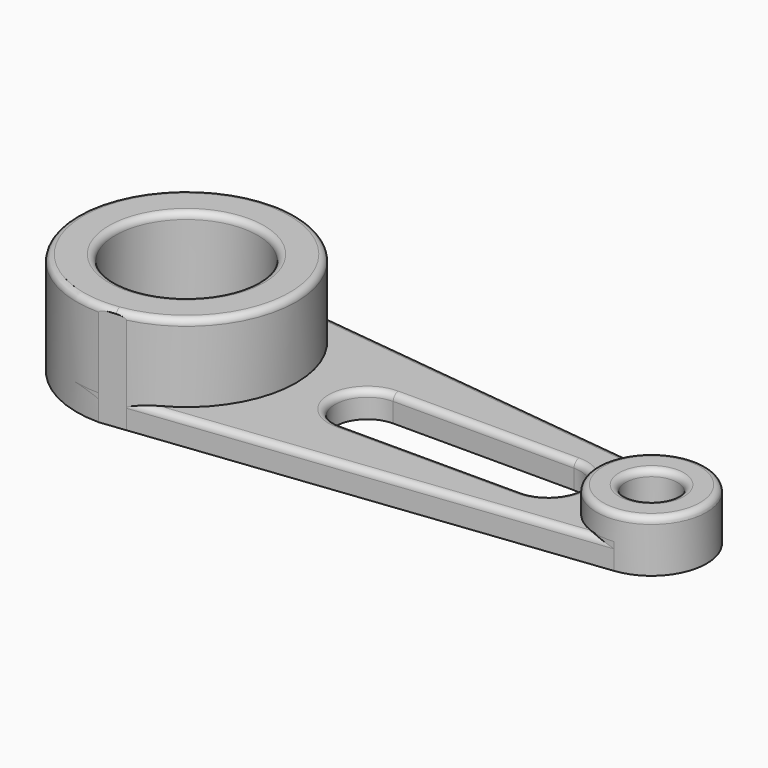
from build123d import *

# Parameters (mm, degrees)
F0_R         = 34.925
F1_DEPTH     = 50.8
F2_DEPTH     = 12.7
F0_R_2       = 12.7
F3_DEPTH     = 25.4
F4_T2_ANGLE  = 196.8788005765
F4_T6_DEPTH  = 273.9624836944
F4_S7_R      = 53.975
F4_T8_DEPTH  = 139
F4_S9_R      = 27.051
F4_T10_DEPTH = 139
F4_T14_DEPTH = 273.9624836944
F4_S15_R     = 53.975
F4_T16_DEPTH = 139
F4_S17_R     = 27.051
F4_T18_DEPTH = 139
F5_R         = 3.174


# Not quite as in the source:
# - a fillet or chamfer that OpenCascade refuses, or shapes differently, is made with other operations: its cross-section is extruded or revolved along the edge and cut away or added
# - a fillet or chamfer is up to 0.001 mm smaller than in the source, because OpenCascade refuses the exact size


with BuildPart() as f1:
    # F0 (on Top) → F1 (new body)
    with BuildSketch(Plane.XY):
        with BuildLine():
            Line((12.4565854601, 52.5179407791), (0, 53.975))
            ThreePointArc((0, 53.975), (-53.975, 0), (0, -53.975))
            Line((0, -53.975), (12.4565854601, -52.5179407791))
            ThreePointArc((12.4565854601, -52.5179407791), (42.3417336986, -33.4735449631), (53.975, 0))
            ThreePointArc((53.975, 0), (42.3417336986, 33.4735449631), (12.4565854601, 52.5179407791))
        make_face()
        Circle(F0_R, mode=Mode.SUBTRACT)
    extrude(amount=F1_DEPTH)

    # F0 (on Top) → F2 (join)
    with BuildSketch(Plane.XY):
        with BuildLine():
            Line((231.7427555563, 26.8678188269), (12.4565854601, 52.5179407791))
            ThreePointArc((12.4565854601, 52.5179407791), (42.3417336986, 33.4735449631), (53.975, 0))
            ThreePointArc((53.975, 0), (42.3417336986, -33.4735449631), (12.4565854601, -52.5179407791))
            Line((12.4565854601, -52.5179407791), (231.7427555563, -26.8678188269))
            ThreePointArc((231.7427555563, -26.8678188269), (201.549, 0), (231.7427555563, 26.8678188269))
        make_face()
        with BuildLine():
            ThreePointArc((88.9, -15.875), (73.025, 0), (88.9, 15.875))
            Line((88.9, 15.875), (177.8, 15.875))
            ThreePointArc((177.8, 15.875), (193.675, 0), (177.8, -15.875))
            Line((177.8, -15.875), (88.9, -15.875))
        make_face(mode=Mode.SUBTRACT)
    extrude(amount=F2_DEPTH)

    # F0 (on Top) → F3 (join)
    with BuildSketch(Plane.XY):
        with BuildLine():
            ThreePointArc((255.651, 0), (248.8085536538, 17.9825181836), (231.7427555563, 26.8678188269))
            ThreePointArc((231.7427555563, 26.8678188269), (201.549, 0), (231.7427555563, -26.8678188269))
            ThreePointArc((231.7427555563, -26.8678188269), (248.8085536538, -17.9825181836), (255.651, 0))
        make_face()
        with Locations((228.6, 0)):
            Circle(F0_R_2, mode=Mode.SUBTRACT)
    extrude(amount=F3_DEPTH)

    # F4: fillet of radius 3.175 on 4 edges, made by hand

    # F4_s1 → F4_t2 (revolve, cut)
    with BuildSketch(Plane(origin=(0, 0, 0), x_dir=(0, 0, 1), z_dir=(0.9891716429, -0.1467632817, 0))):
        with BuildLine():
            ThreePointArc((50.8, -50.8), (49.8700640303, -53.0450640303), (47.625, -53.975))
            Line((47.625, -53.975), (50.8, -53.975))
            Line((50.8, -53.975), (50.8, -50.8))
        make_face()
    revolve(axis=Axis((0, 0, 50.8), (0, 0, 1)), revolution_arc=F4_T2_ANGLE, mode=Mode.SUBTRACT)


with BuildPart() as f4_tool4:
    # F4_s5 → F4_t6 (new body)
    with BuildSketch(Plane(origin=(238.9168372411, -27.9463406606, 0), x_dir=(0, 0, 1), z_dir=(-0.9932283031, 0.1161789049, 0))):
        with BuildLine():
            ThreePointArc((9.525, 53.6094976592), (11.7700640303, 52.6795616895), (12.7, 50.4344976592))
            Line((12.7, 50.4344976592), (12.7, 53.6094976592))
            Line((12.7, 53.6094976592), (9.525, 53.6094976592))
        make_face()
    extrude(amount=F4_T6_DEPTH)

    # F4_s7 → F4_t8 (cut, symmetric)
    with BuildSketch(Plane.XY.offset(11.1)):
        Circle(F4_S7_R)
    extrude(amount=F4_T8_DEPTH, both=True, mode=Mode.SUBTRACT)

    # F4_s9 → F4_t10 (cut, symmetric)
    with BuildSketch(Plane.XY.offset(11.1)):
        with Locations((228.6, 0)):
            Circle(F4_S9_R)
    extrude(amount=F4_T10_DEPTH, both=True, mode=Mode.SUBTRACT)


with BuildPart() as f1_1:
    add(f1.part)

    # F4_t3: cut F4_tool4
    add(f4_tool4.part, mode=Mode.SUBTRACT)


with BuildPart() as f4_tool12:
    # F4_s13 → F4_t14 (new body)
    with BuildSketch(Plane(origin=(-33.1904555488, -3.8823206776, 0), x_dir=(0, 0, 1), z_dir=(0.9932283031, 0.1161789049, 0))):
        with BuildLine():
            ThreePointArc((12.7, 50.4344976592), (11.7700640303, 52.6795616895), (9.525, 53.6094976592))
            Line((9.525, 53.6094976592), (12.7, 53.6094976592))
            Line((12.7, 53.6094976592), (12.7, 50.4344976592))
        make_face()
    extrude(amount=F4_T14_DEPTH)

    # F4_s15 → F4_t16 (cut, symmetric)
    with BuildSketch(Plane.XY.offset(11.1)):
        Circle(F4_S15_R)
    extrude(amount=F4_T16_DEPTH, both=True, mode=Mode.SUBTRACT)

    # F4_s17 → F4_t18 (cut, symmetric)
    with BuildSketch(Plane.XY.offset(11.1)):
        with Locations((228.6, 0)):
            Circle(F4_S17_R)
    extrude(amount=F4_T18_DEPTH, both=True, mode=Mode.SUBTRACT)


with BuildPart() as f1_2:
    add(f1_1.part)

    # F4_t11: cut F4_tool12
    add(f4_tool12.part, mode=Mode.SUBTRACT)

    # F4_s19 → F4_t20 (revolve, cut)
    with BuildSketch(Plane(origin=(225.5144628263, 26.3786515627, 0), x_dir=(0, 0, 1), z_dir=(0.9932283031, 0.1161789049, 0))):
        with BuildLine():
            ThreePointArc((22.225, 53.6094976592), (24.4700640303, 52.6795616895), (25.4, 50.4344976592))
            Line((25.4, 50.4344976592), (25.4, 53.6094976592))
            Line((25.4, 53.6094976592), (22.225, 53.6094976592))
        make_face()
    revolve(axis=Axis((228.6, 0, 25.4), (0, 0, -1)), mode=Mode.SUBTRACT)

    # F5 (radius 3.175 in the source; OpenCascade refuses exactly that, so slightly less here)
    f5_edges = [f1_2.edges().sort_by_distance(p)[0] for p in [
        (-34.925, 0, 50.8),
        (133.35, 15.875, 12.7),
        (215.9, 0, 25.4),
        (73.025, 0, 12.7),
        (133.35, -15.875, 12.7),
        (193.675, 0, 12.7),
        (53.975, 0, 50.8),
    ]]
    fillet(f5_edges, radius=F5_R)


solid = f1_2.part
